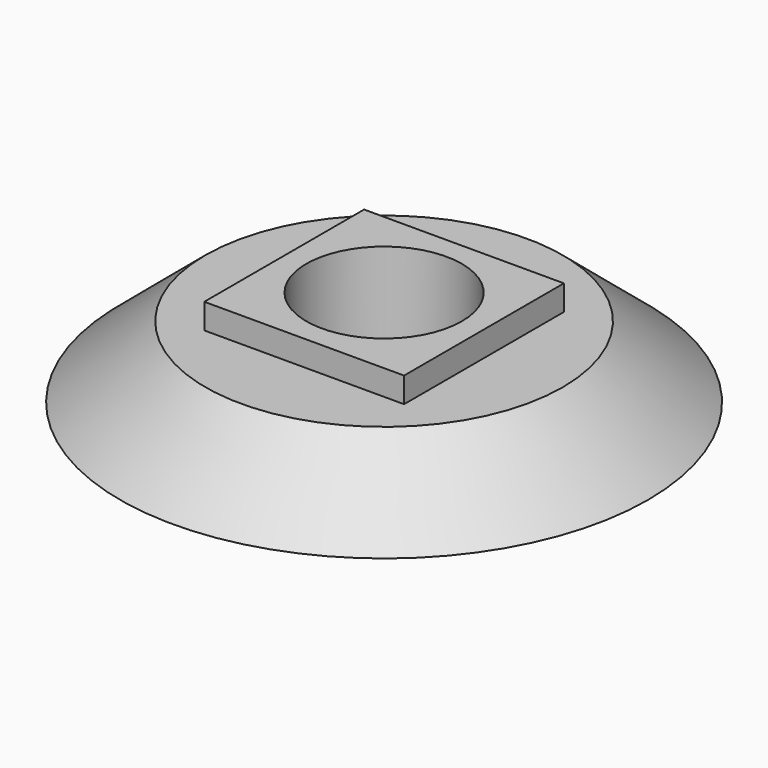
from build123d import *

# Parameters (mm, degrees)
F0_R     = 14
F0_W     = 9.5
F0_H     = 9.5
F1_DEPTH = 3.4
F0_R_2   = 3.7
F2_DEPTH = 4.6


# Not quite as in the source:
# - a fillet or chamfer that OpenCascade refuses, or shapes differently, is made with other operations: its cross-section is extruded or revolved along the edge and cut away or added


with BuildPart() as f1:
    # F0 (on Top) → F1 (new body)
    with BuildSketch(Plane.XY):
        Circle(F0_R)
        Rectangle(F0_W, F0_H, mode=Mode.SUBTRACT)
    extrude(amount=F1_DEPTH)

    # F0 (on Top) → F2 (join)
    with BuildSketch(Plane.XY):
        Rectangle(F0_W, F0_H)
        Circle(F0_R_2, mode=Mode.SUBTRACT)
    extrude(amount=F2_DEPTH)

    # F3: chamfer of 5.5 x 4.6150479715 on 1 edges, made by hand

    # F3_s1 → F3_t2 (revolve, cut)
    with BuildSketch(Plane.XZ):
        Polygon((14, -1.2150479715), (8.5, 3.4), (14, 3.4), align=None)
    revolve(axis=Axis((0, 0, 3.4), (0, 0, 1)), mode=Mode.SUBTRACT)


solid = f1.part
